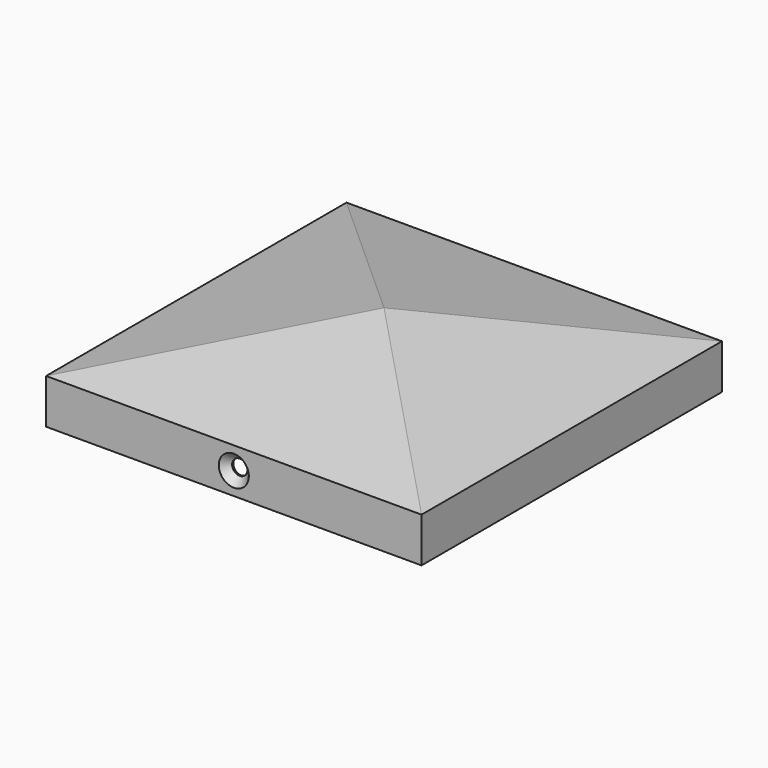
from build123d import *

# Parameters (mm, degrees)
F0_W            = 84
F0_H            = 84
F1_DEPTH        = 10
F2_W            = 80
F2_H            = 80
F3_DEPTH        = 9.5
F4_W            = 84
F4_H            = 84
F5_DEPTH        = 10
F6_SIZE2        = 9.99999
F6_SIZE         = 41.99999
F8_D            = 3.4
F8_DEPTH        = 12
F8_CSINK_D      = 6.72
F8_CSINK_ANGLE  = 90
F8_TIP          = 1.0214630523
F10_D           = 3.4
F10_DEPTH       = 12
F10_CSINK_D     = 6.72
F10_CSINK_ANGLE = 90
F10_TIP         = 1.0214630523


# Not quite as in the source:
# - a fillet or chamfer is up to 0.001 mm smaller than in the source, because OpenCascade refuses the exact size


with BuildPart() as f1:
    # F0 (on Top) → F1 (new body)
    with BuildSketch(Plane.XY):
        with Locations((42, 42)):
            Rectangle(F0_W, F0_H)
    extrude(amount=F1_DEPTH)

    # F2 (on face) → F3 (cut)
    with BuildSketch(Plane(origin=(0, 0, 0), x_dir=(1, 0, 0), z_dir=(0, 0, -1))):
        with Locations((42, -42)):
            Rectangle(F2_W, F2_H)
    extrude(amount=-F3_DEPTH, mode=Mode.SUBTRACT)

    # F4 (on face) → F5 (join)
    with BuildSketch(Plane.XY.offset(10)):
        with Locations((42, 42)):
            Rectangle(F4_W, F4_H)
    extrude(amount=F5_DEPTH)

    # F6 (size 42 and 10 in the source; OpenCascade refuses exactly that, so slightly less here)
    f6_edges = [f1.edges().sort_by_distance(p)[0] for p in [
        (0, 42, 20),
        (42, 84, 20),
        (84, 42, 20),
        (42, 0, 20),
    ]]
    f6_side = f1.faces().sort_by_distance((42, 42, 20))[0]
    chamfer(f6_edges, length=F6_SIZE, length2=F6_SIZE2, reference=f6_side)

    # F8
    with Locations(Plane.XZ):
        with Locations((42, 5)):
            CounterSinkHole(F8_D / 2, F8_CSINK_D / 2, depth=F8_DEPTH, counter_sink_angle=F8_CSINK_ANGLE)
            with Locations((0, 0, -(F8_DEPTH + F8_TIP / 2))):  # 118° drill point
                Cone(0, F8_D / 2, F8_TIP, mode=Mode.SUBTRACT)

    # F10
    with Locations(Plane(origin=(0, 84, 0), x_dir=(-1, 0, 0), z_dir=(0, 1, 0))):
        with Locations((-42, 5)):
            CounterSinkHole(F10_D / 2, F10_CSINK_D / 2, depth=F10_DEPTH, counter_sink_angle=F10_CSINK_ANGLE)
            with Locations((0, 0, -(F10_DEPTH + F10_TIP / 2))):  # 118° drill point
                Cone(0, F10_D / 2, F10_TIP, mode=Mode.SUBTRACT)


solid = f1.part
